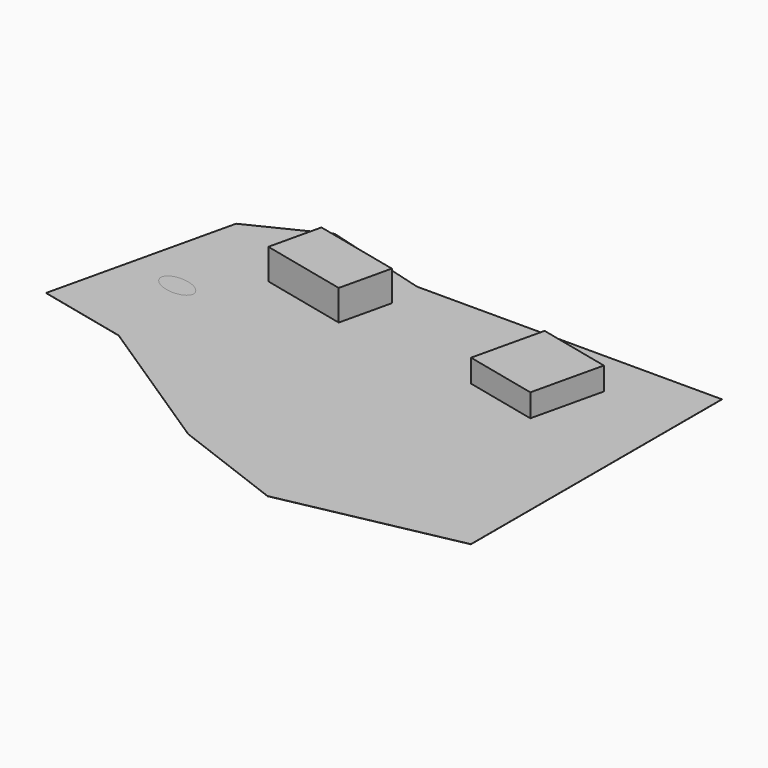
from build123d import *

# Parameters (mm, degrees)
F1_DEPTH = 25.4
F2_DEPTH = 6096
F3_DEPTH = 4572
F4_DEPTH = 25.4
F5_DEPTH = 25.4


# Not quite as in the source:
# - a feature names something its author has since deleted; it is built from what else it names


with BuildPart() as f1:
    # F0 (on Top) → F1 (new body)
    with BuildSketch(Plane.XY):
        Polygon((-33112.4640655049, -3647.3720976521), (-1.6886040407, 3110.491777778), (-1.6886040407, 62737.1229546988), (-60961.6886040408, 62737.1229546987), (-82155.8610464841, 68661.2885088993), (-96316.7696711288, 61713.7123499455), (-104438.0283558496, 26676.2026448331), (-86304.1977238219, 22473.00640182), (-56902.1438828347, 3159.4669638971), (-36770.0640655049, -4481.2923027159), (-36770.0640655049, -599.3720976521), (-33112.4640655049, -599.3720976521), align=None)
        with BuildLine():
            add(Edge.make_bspline(
                [(-94128.4642083729, 40489.2396473104), (-94962.9136036562, 36889.1783857883), (-88978.2879994819, 37398.7547763924), (-82993.6623953076, 37908.3311669965), (-88143.8386041986, 40998.8160379144), (-93294.0148130897, 44089.3009088324), (-94128.4642083729, 40489.2396473104)],
                knots=[0, 0, 0, 2.0943951024, 2.0943951024, 4.1887902048, 4.1887902048, 6.2831853072, 6.2831853072, 6.2831853072], degree=2, weights=[1, 0.5, 1, 0.5, 1, 0.5, 1]))
        make_face(mode=Mode.SUBTRACT)
        Polygon((-80191.2308576593, 49617.5479871827), (-77805.3243514137, 59911.0536632609), (-60534.0095391478, 55907.7778426853), (-62919.9160453934, 45614.272166607), align=None, mode=Mode.SUBTRACT)
        Polygon((-33888.8404387287, 42397.5516428327), (-30585.277583927, 56650.0979635563), (-16035.8032148549, 53277.7108826129), (-19339.3660696566, 39025.1645618892), align=None, mode=Mode.SUBTRACT)
        Polygon((-34941.264065505, -7131.4640898385), (0, 0), (-1.6886040407, 9.2829546987), (-1.6886040407, 3110.491777778), (-33112.4640655049, -3647.3720976521), (-33112.4640655049, -599.3720976521), (-36770.0640655049, -599.3720976521), (-36770.0640655049, -4481.2923027159), (-56902.1438828347, 3159.4669638971), (-86304.1977238219, 22473.00640182), (-104438.0283558496, 26676.2026448331), (-104850.9737126999, 24894.6343547425), (-87035.2908096331, 20765.1807955688), (-57738.5711688761, 1520.832994438), align=None)
        Polygon((-16035.8032148549, 53277.7108826129), (-30585.277583927, 56650.0979635563), (-33888.8404387287, 42397.5516428327), (-19339.3660696566, 39025.1645618892), align=None)
        Polygon((-60534.0095391478, 55907.7778426853), (-77805.3243514137, 59911.0536632609), (-80191.2308576593, 49617.5479871827), (-62919.9160453935, 45614.272166607), align=None)
    extrude(amount=-F1_DEPTH)

    # F0 (on Top) → F4 (cut, through all)
    with BuildSketch(Plane.XY):
        with BuildLine():
            add(Edge.make_bspline(
                [(-94128.4642083729, 40489.2396473104), (-94962.9136036562, 36889.1783857883), (-88978.2879994819, 37398.7547763924), (-82993.6623953076, 37908.3311669965), (-88143.8386041986, 40998.8160379144), (-93294.0148130897, 44089.3009088324), (-94128.4642083729, 40489.2396473104)],
                knots=[0, 0, 0, 2.0943951024, 2.0943951024, 4.1887902048, 4.1887902048, 6.2831853072, 6.2831853072, 6.2831853072], degree=2, weights=[1, 0.5, 1, 0.5, 1, 0.5, 1]))
        make_face()
    extrude(amount=-F4_DEPTH, mode=Mode.SUBTRACT)


with BuildPart() as f2:
    # F0 (on Top) → F2 (new body)
    with BuildSketch(Plane.XY):
        Polygon((-60534.0095391478, 55907.7778426853), (-77805.3243514137, 59911.0536632609), (-80191.2308576593, 49617.5479871827), (-62919.9160453935, 45614.272166607), align=None)
    extrude(amount=F2_DEPTH)


with BuildPart() as f3:
    # F0 (on Top) → F3 (new body)
    with BuildSketch(Plane.XY):
        Polygon((-16035.8032148549, 53277.7108826129), (-30585.277583927, 56650.0979635563), (-33888.8404387287, 42397.5516428327), (-19339.3660696566, 39025.1645618892), align=None)
    extrude(amount=F3_DEPTH)


with BuildPart() as f5:
    # F0 (on Top) → F5 (new body, through all)
    with BuildSketch(Plane.XY):
        with BuildLine():
            add(Edge.make_bspline(
                [(-94128.4642083729, 40489.2396473104), (-94962.9136036562, 36889.1783857883), (-88978.2879994819, 37398.7547763924), (-82993.6623953076, 37908.3311669965), (-88143.8386041986, 40998.8160379144), (-93294.0148130897, 44089.3009088324), (-94128.4642083729, 40489.2396473104)],
                knots=[0, 0, 0, 2.0943951024, 2.0943951024, 4.1887902048, 4.1887902048, 6.2831853072, 6.2831853072, 6.2831853072], degree=2, weights=[1, 0.5, 1, 0.5, 1, 0.5, 1]))
        make_face()
    extrude(amount=-F5_DEPTH)


solid = Compound([f1.part, f2.part, f3.part, f5.part])
